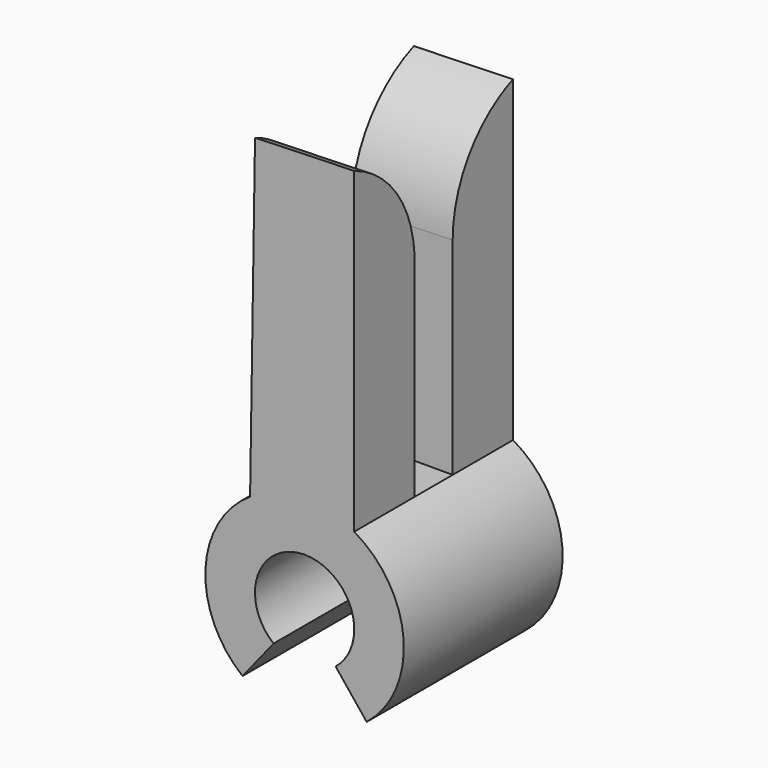
from build123d import *

# Parameters (mm, degrees)
F1_DEPTH    = 6.35
F2_W        = 1.524
F2_H        = 10.16
F3_DEPTH    = 25.4
F4_T1_DEPTH = 20.8982128859
F5_T1_DEPTH = 20.8982128859


# Not quite as in the source:
# - a fillet or chamfer that OpenCascade refuses, or shapes differently, is made with other operations: its cross-section is extruded or revolved along the edge and cut away or added


with BuildPart() as f1:
    # F0 (on Front) → F1 (new body)
    with BuildSketch(Plane.XZ):
        with BuildLine():
            Line((0.9929372138, -1.2386411666), (1.9858744275, -2.4772823331))
            ThreePointArc((1.9858744275, -2.4772823331), (3.1658183857, 0.2412860305), (1.5875, 2.749630657))
            Line((1.5875, 2.749630657), (1.5875, 12.909630657))
            Line((1.5875, 12.909630657), (-1.58600151, 12.8120951952))
            Line((-1.58600151, 12.8120951952), (-1.7437092207, 2.653319271))
            ThreePointArc((-1.7437092207, 2.653319271), (-3.1714691788, 0.1496938466), (-1.9858744275, -2.4772823331))
            Line((-1.9858744275, -2.4772823331), (-0.9929372138, -1.2386411666))
            ThreePointArc((-0.9929372138, -1.2386411666), (0, 1.5875), (0.9929372138, -1.2386411666))
        make_face()
    extrude(amount=F1_DEPTH)

    # F2 (on face) → F3 (cut)
    with BuildSketch(Plane.YZ.offset(1.5875)):
        with Locations((-3.175, 7.829630657)):
            Rectangle(F2_W, F2_H)
    extrude(amount=-F3_DEPTH, mode=Mode.SUBTRACT)

    # F4: fillet of radius 3.81 on 1 edges, made by hand

    # F4_s2 → F4_t1 (cut)
    with BuildSketch(Plane(origin=(10.839820428, 0, 0.3331546837), x_dir=(0, 1, 0), z_dir=(-0.9995280346, 0, -0.0307198305))):
        with BuildLine():
            ThreePointArc((-6.35, -12.8547700275), (-4.597502421, -11.4541342134), (-3.937, -9.3101274503))
            Line((-3.937, -9.3101274503), (-3.937, -12.8547700275))
            Line((-3.937, -12.8547700275), (-6.35, -12.8547700275))
        make_face()
    extrude(amount=F4_T1_DEPTH, mode=Mode.SUBTRACT)

    # F5: fillet of radius 3.81 on 1 edges, made by hand

    # F5_s2 → F5_t1 (cut)
    with BuildSketch(Plane(origin=(-10.0485292251, 0, -0.308834874), x_dir=(0, 1, 0), z_dir=(0.9995280346, 0, 0.0307198305))):
        with BuildLine():
            ThreePointArc((0, 12.8547700275), (-1.752497579, 11.4541342134), (-2.413, 9.3101274503))
            Line((-2.413, 9.3101274503), (-2.413, 12.8547700275))
            Line((-2.413, 12.8547700275), (0, 12.8547700275))
        make_face()
    extrude(amount=F5_T1_DEPTH, mode=Mode.SUBTRACT)


solid = f1.part
